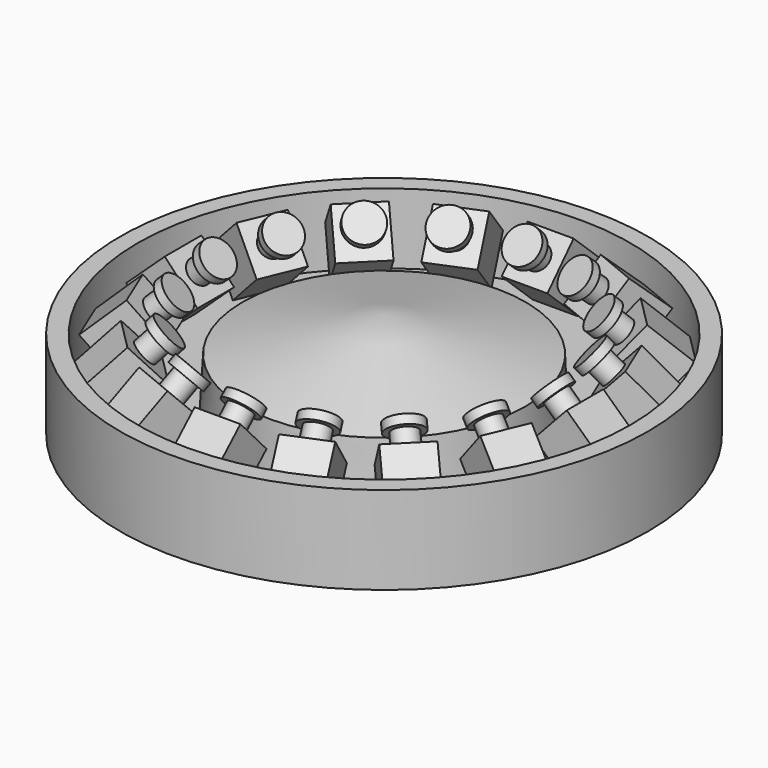
from build123d import *

# Parameters (mm, degrees)
F0_R      = 150
F1_DEPTH  = 50
F2_T      = -10
F7_W      = 26.0129887611
F7_H      = 27.2390077947
F8_DEPTH  = 30
F9_R      = 6.9386007548
F10_DEPTH = 10
F11_R     = 10.1905415086
F11_R_2   = 6.9386007548
F12_DEPTH = 5
F13_COUNT = 16


# Not quite as in the source:
# - the program builds the solid bodies; features that only make, move or delete a surface that nothing else refers to are left out


with BuildPart() as f1:
    # F0 (on Top) → F1 (new body)
    with BuildSketch(Plane.XY):
        Circle(F0_R)
    extrude(amount=F1_DEPTH)

    # F2
    f2_openings = [f1.faces().sort_by_distance(p)[0] for p in [
        (0, 0, 50),
    ]]
    offset(amount=F2_T, openings=f2_openings)


with BuildPart() as f8:
    # F7 (on face) → F8 (new body)
    with BuildSketch(Plane(origin=(-56.2995517793, 0, -52.4018876703), x_dir=(0, -1, 0), z_dir=(-0.7319908191, 0, -0.6813144948))):
        with Locations((-2.0171441138, 105.9626182138)):
            Rectangle(F7_W, F7_H)
    extrude(amount=-F8_DEPTH)

    # F9 (on face) → F10 (join)
    with BuildSketch(Plane(origin=(-34.3398272072, 0, -31.962452827), x_dir=(0, 1, 0), z_dir=(0.7319908191, 0, 0.6813144948))):
        with Locations((1.7930696486, 106.2461510301)):
            Circle(F9_R)
    extrude(amount=F10_DEPTH)

    # F11 (on face) → F12 (join)
    with BuildSketch(Plane(origin=(-27.0199190164, 0, -25.1493078792), x_dir=(0, 1, 0), z_dir=(0.7319908191, 0, 0.6813144948))):
        with Locations((1.7930696486, 106.2461510301)):
            Circle(F11_R)
        with Locations((1.7930696486, 106.2461510301)):
            Circle(F11_R_2, mode=Mode.SUBTRACT)
        with Locations((1.7930696486, 106.2461510301)):
            Circle(F11_R_2)
    extrude(amount=F12_DEPTH)


with BuildPart() as f13_1:
    # F13: instance of F8
    add(f8.part.rotate(Axis((0, 0, 79.5852057636), (0, 0, -1)), 1 * 360 / F13_COUNT))


with BuildPart() as f13_2:
    # F13: instance of F8
    add(f8.part.rotate(Axis((0, 0, 79.5852057636), (0, 0, -1)), 2 * 360 / F13_COUNT))


with BuildPart() as f13_3:
    # F13: instance of F8
    add(f8.part.rotate(Axis((0, 0, 79.5852057636), (0, 0, -1)), 3 * 360 / F13_COUNT))


with BuildPart() as f13_4:
    # F13: instance of F8
    add(f8.part.rotate(Axis((0, 0, 79.5852057636), (0, 0, -1)), 4 * 360 / F13_COUNT))


with BuildPart() as f13_5:
    # F13: instance of F8
    add(f8.part.rotate(Axis((0, 0, 79.5852057636), (0, 0, -1)), 5 * 360 / F13_COUNT))


with BuildPart() as f13_6:
    # F13: instance of F8
    add(f8.part.rotate(Axis((0, 0, 79.5852057636), (0, 0, -1)), 6 * 360 / F13_COUNT))


with BuildPart() as f13_7:
    # F13: instance of F8
    add(f8.part.rotate(Axis((0, 0, 79.5852057636), (0, 0, -1)), 7 * 360 / F13_COUNT))


with BuildPart() as f13_8:
    # F13: instance of F8
    add(f8.part.rotate(Axis((0, 0, 79.5852057636), (0, 0, -1)), 8 * 360 / F13_COUNT))


with BuildPart() as f13_9:
    # F13: instance of F8
    add(f8.part.rotate(Axis((0, 0, 79.5852057636), (0, 0, -1)), 9 * 360 / F13_COUNT))


with BuildPart() as f13_10:
    # F13: instance of F8
    add(f8.part.rotate(Axis((0, 0, 79.5852057636), (0, 0, -1)), 10 * 360 / F13_COUNT))


with BuildPart() as f13_11:
    # F13: instance of F8
    add(f8.part.rotate(Axis((0, 0, 79.5852057636), (0, 0, -1)), 11 * 360 / F13_COUNT))


with BuildPart() as f13_12:
    # F13: instance of F8
    add(f8.part.rotate(Axis((0, 0, 79.5852057636), (0, 0, -1)), 12 * 360 / F13_COUNT))


with BuildPart() as f13_13:
    # F13: instance of F8
    add(f8.part.rotate(Axis((0, 0, 79.5852057636), (0, 0, -1)), 13 * 360 / F13_COUNT))


with BuildPart() as f13_14:
    # F13: instance of F8
    add(f8.part.rotate(Axis((0, 0, 79.5852057636), (0, 0, -1)), 14 * 360 / F13_COUNT))


with BuildPart() as f13_15:
    # F13: instance of F8
    add(f8.part.rotate(Axis((0, 0, 79.5852057636), (0, 0, -1)), 15 * 360 / F13_COUNT))


with BuildPart() as f15:
    # F14 (on Front) → F15 (revolve)
    with BuildSketch(Plane.XZ):
        Polygon((-80.3637504578, 39.8807749152), (-81.9754377007, 10.1797431707), (0, 10.4099847376), (0, 59.6814639866), align=None)
    revolve(axis=Axis((0, 0, 35.0457243621), (0, 0, -1)))


solid = Compound([f1.part, f8.part, f13_1.part, f13_2.part, f13_3.part, f13_4.part, f13_5.part, f13_6.part, f13_7.part, f13_8.part, f13_9.part, f13_10.part, f13_11.part, f13_12.part, f13_13.part, f13_14.part, f13_15.part, f15.part])
